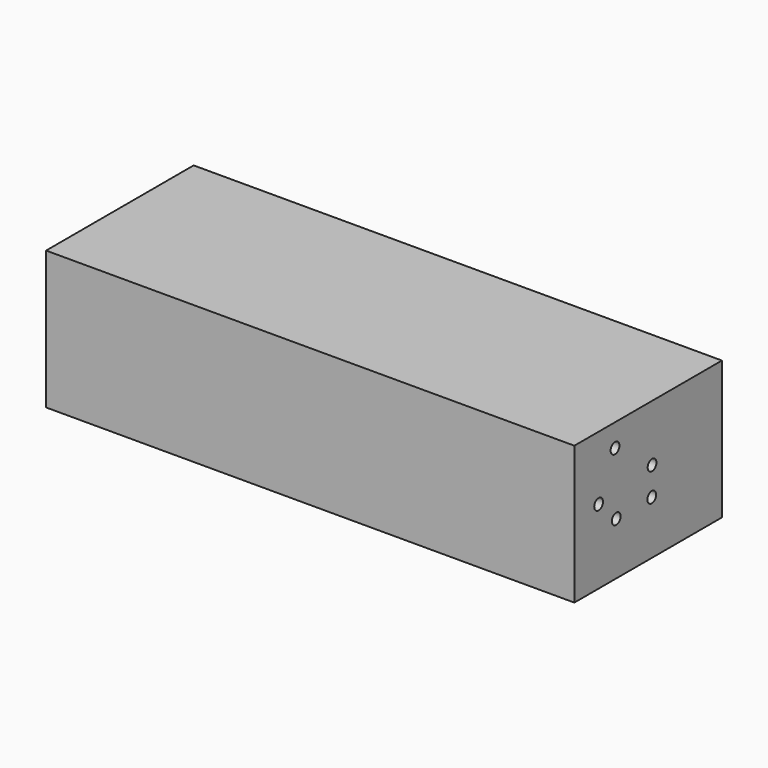
from build123d import *

# Parameters (mm, degrees)
F0_W     = 122.3997175694
F0_H     = 42.7361652255
F1_DEPTH = 32.0060774684
F5_D     = 2.54


# Not quite as in the source:
# - the program builds the solid bodies; features that only make, move or delete a surface that nothing else refers to are left out


with BuildPart() as f1:
    # F0 (on Top) → F1 (new body)
    with BuildSketch(Plane.XY):
        with Locations((-1.4522224665, 37.9646681249)):
            Rectangle(F0_W, F0_H)
    extrude(amount=F1_DEPTH)

    # F5 (through all)
    with Locations(Plane(origin=(-62.6520812511, 0, 0), x_dir=(0, -1, 0), z_dir=(-1, 0, 0))):
        with Locations((-28.3709894866, 26.730036363), (-23.6220490187, 17.2120258212), (-28.7239328027, 12.1772345155), (-39.0075407922, 12.403704226), (-39.0968136489, 18.9130250365)):
            Hole(F5_D / 2)


solid = f1.part
